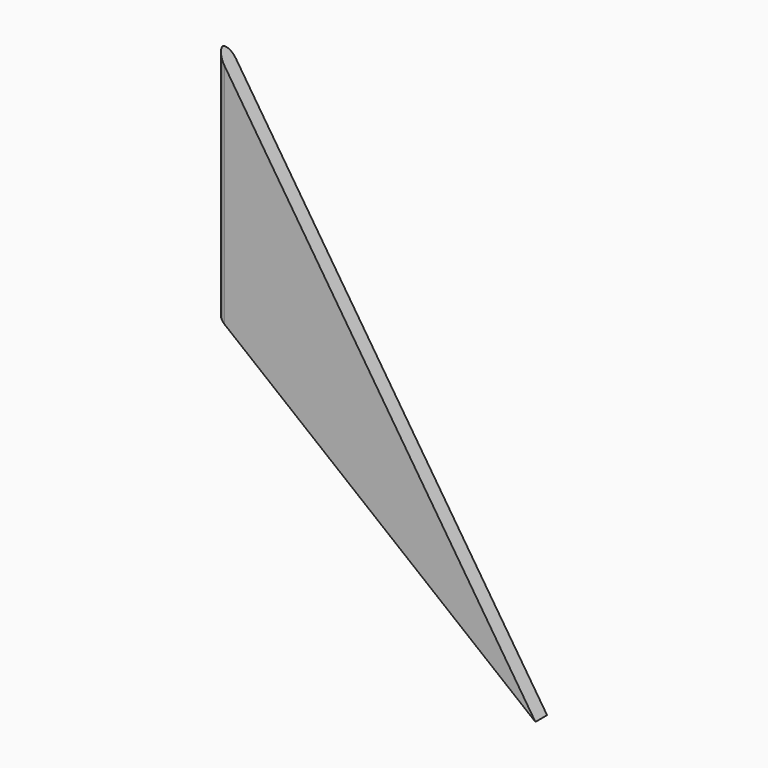
from build123d import *

# Parameters (mm, degrees)
F1_DEPTH    = 2.5
F2_T1_DEPTH = 46.7597979746


# Not quite as in the source:
# - a fillet or chamfer that OpenCascade refuses, or shapes differently, is made with other operations: its cross-section is extruded or revolved along the edge and cut away or added


with BuildPart() as f1:
    # F0 (on Front) → F1 (new body)
    with BuildSketch(Plane.XZ):
        Polygon((0, 40), (0, 0), (54.643732486, -43.75), align=None)
    extrude(amount=F1_DEPTH)

    # F2: fillet of radius 1.3519595949 on 2 edges, made by hand

    # F2_s2 → F2_t1 (cut)
    with BuildSketch(Plane.XY.offset(-3.3798989873)):
        with BuildLine():
            ThreePointArc((0, -1.1480404051), (0.3959797975, -2.1040202025), (1.3519595949, -2.5))
            Line((1.3519595949, -2.5), (0, -2.5))
            Line((0, -2.5), (0, -1.1480404051))
        make_face()
        with BuildLine():
            ThreePointArc((0, -1.3519595949), (0.3959797975, -0.3959797975), (1.3519595949, 0))
            Line((1.3519595949, 0), (0, 0))
            Line((0, 0), (0, -1.3519595949))
        make_face()
    extrude(amount=F2_T1_DEPTH, mode=Mode.SUBTRACT)


solid = f1.part
